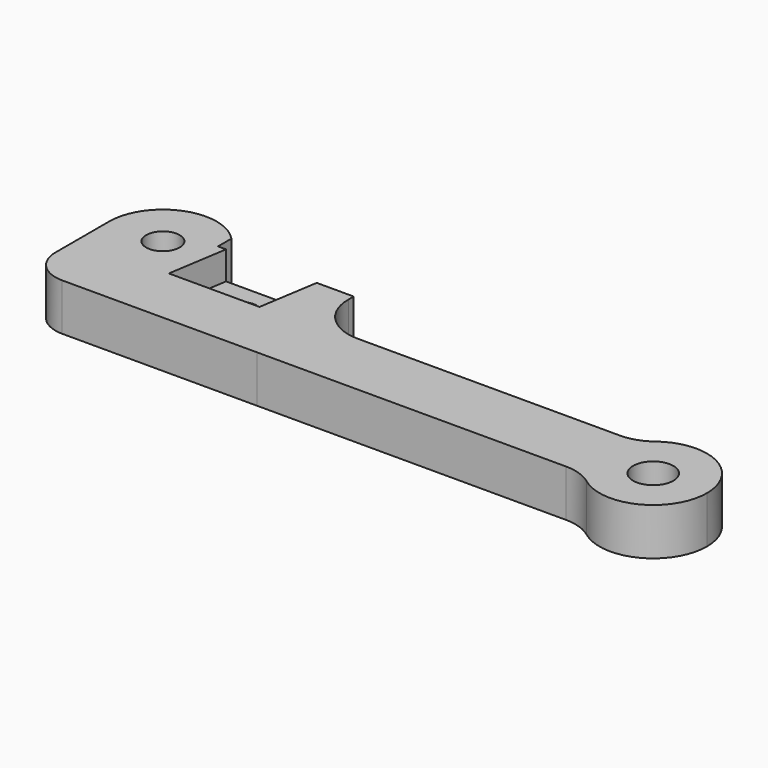
from build123d import *

# Parameters (mm, degrees)
F1_DEPTH    = 7
F2_R        = 2
F3_DEPTH    = 4.2
F4_DEPTH    = 25
F5_R        = 2.5
F6_DEPTH    = 25
F7_R        = 8
F8_R        = 5
F9_T1_DEPTH = 52
F11_DEPTH   = 25
F13_DEPTH   = 25
F14_R       = 3
F15_DEPTH   = 25
F16_R       = 7


# Not quite as in the source:
# - a fillet or chamfer that OpenCascade refuses, or shapes differently, is made with other operations: its cross-section is extruded or revolved along the edge and cut away or added
# - ends of sketch curves that miss each other by under 0.0002 mm in the source are joined
# - a feature names something its author has since deleted; it is built from what else it names


with BuildPart() as f1:
    # F0 (on Top) → F1 (new body)
    with BuildSketch(Plane.XY):
        Polygon((-2, 17), (-17.0000004771, 17), (-16.9999997194, -10.0000004771), (17.0000002806, -9.9999995229), (17, 4.771e-07), (16.9999997755, 8), (-2, 8), align=None)
        with BuildLine():
            Line((17, 4.771e-07), (17.0000002806, -9.9999995229))
            Line((17.0000002806, -9.9999995229), (65.7550022822, -9.9999995229))
            ThreePointArc((65.7550022822, -9.9999995229), (64.0000002806, -4.9999995229), (65.7550022822, 4.771e-07))
            Line((65.7550022822, 4.771e-07), (17, 4.771e-07))
        make_face()
        with BuildLine():
            ThreePointArc((65.7550022822, 4.771e-07), (64.0000002806, -4.9999995229), (65.7550022822, -9.9999995229))
            Line((65.7550022822, -9.9999995229), (72.0000002806, -9.9999995229))
            Line((72.0000002806, -9.9999995229), (72.0000002806, 4.771e-07))
            Line((72.0000002806, 4.771e-07), (65.7550022822, 4.771e-07))
        make_face()
        with BuildLine():
            Line((72.0000002806, -9.9999995229), (65.7550022822, -9.9999995229))
            ThreePointArc((65.7550022822, -9.9999995229), (74.6495300514, -12.5485087793), (80.0000002806, -4.9999995229))
            ThreePointArc((80.0000002806, -4.9999995229), (74.6495300514, 2.5485097334), (65.7550022822, 4.771e-07))
            Line((65.7550022822, 4.771e-07), (72.0000002806, 4.771e-07))
            Line((72.0000002806, 4.771e-07), (72.0000002806, -9.9999995229))
        make_face()
    extrude(amount=F1_DEPTH)

    # F2 (on face) → F3 (cut)
    with BuildSketch(Plane.XY.offset(7)):
        Polygon((11.5, 8), (-2, 8), (-3.4079101854, -0.8891950654), (10.0920898146, -0.8891950654), align=None)
        with Locations((4.0460449073, 3.5554024673)):
            Circle(F2_R, mode=Mode.SUBTRACT)
    extrude(amount=-F3_DEPTH, mode=Mode.SUBTRACT)

    # F4 (cut): a face of the model
    f4_faces = [f1.faces().sort_by_distance(p)[0] for p in [
        (4.0460449073, 3.5554024673, 7),
    ]]
    extrude(f4_faces, amount=-F4_DEPTH, mode=Mode.SUBTRACT)

    # F5 (on face) → F6 (cut)
    with BuildSketch(Plane.XY.offset(7)):
        with Locations((-9, 5)):
            Circle(F5_R)
    extrude(amount=-F6_DEPTH, mode=Mode.SUBTRACT)

    # F7
    f7_edges = [f1.edges().sort_by_distance(p)[0] for p in [
        (-17, 17, 3.5),
    ]]
    fillet(f7_edges, radius=F7_R)

    # F8
    f8_edges = [f1.edges().sort_by_distance(p)[0] for p in [
        (-17, -10, 3.5),
    ]]
    fillet(f8_edges, radius=F8_R)

    # F9: fillet of radius 9 on 1 edges, made by hand

    # F9_s2 → F9_t1 (cut)
    with BuildSketch(Plane.XY.offset(-22.5)):
        with BuildLine():
            ThreePointArc((-11, 17), (-4.6360389693, 14.3639610307), (-2, 8))
            Line((-2, 8), (-2, 17))
            Line((-2, 17), (-11, 17))
        make_face()
    extrude(amount=F9_T1_DEPTH, mode=Mode.SUBTRACT)

    # F10 (on face) → F11 (cut)
    with BuildSketch(Plane.XY.offset(7)):
        with BuildLine():
            ThreePointArc((-3.2, 12.4899888642), (-2.3051739523, 10.3237900078), (-2, 8))
            Line((-2, 8), (-2, 18))
            Line((-2, 18), (-3.2, 18))
            Line((-3.2, 18), (-3.2, 12.4899888642))
        make_face()
        with BuildLine():
            Line((-3.2, 8), (-2, 8))
            ThreePointArc((-2, 8), (-2.3051739523, 10.3237900078), (-3.2, 12.4899888642))
            Line((-3.2, 12.4899888642), (-3.2, 8))
        make_face()
    extrude(amount=-F11_DEPTH, mode=Mode.SUBTRACT)

    # F12 (on face) → F13 (cut)
    with BuildSketch(Plane.XY.offset(7)):
        with BuildLine():
            ThreePointArc((-17, 4.9999997208), (-11.9664795245, 12.4296701966), (-3.2, 10.5099909256))
            Line((-3.2, 10.5099909256), (-3.2, 12.4899888642))
            ThreePointArc((-3.2, 12.4899888642), (-6.0560248177, 15.5204460903), (-9.9704600393, 16.9409198335))
            ThreePointArc((-9.9704600393, 16.9409198335), (-14.9901454961, 14.3026559347), (-17.0000002526, 8.9999997755))
            Line((-17.0000002526, 8.9999997755), (-17, 4.9999997208))
        make_face()
    extrude(amount=-F13_DEPTH, mode=Mode.SUBTRACT)

    # F14 (on face) → F15 (cut)
    with BuildSketch(Plane.XY.offset(7)):
        with Locations((72.0000002806, -4.9999995229)):
            Circle(F14_R)
    extrude(amount=-F15_DEPTH, mode=Mode.SUBTRACT)

    # F16
    f16_edges = [f1.edges().sort_by_distance(p)[0] for p in [
        (17, 0, 3.5),
        (65.755002, -10, 3.5),
        (65.755002, 0, 3.5),
    ]]
    fillet(f16_edges, radius=F16_R)


solid = f1.part
